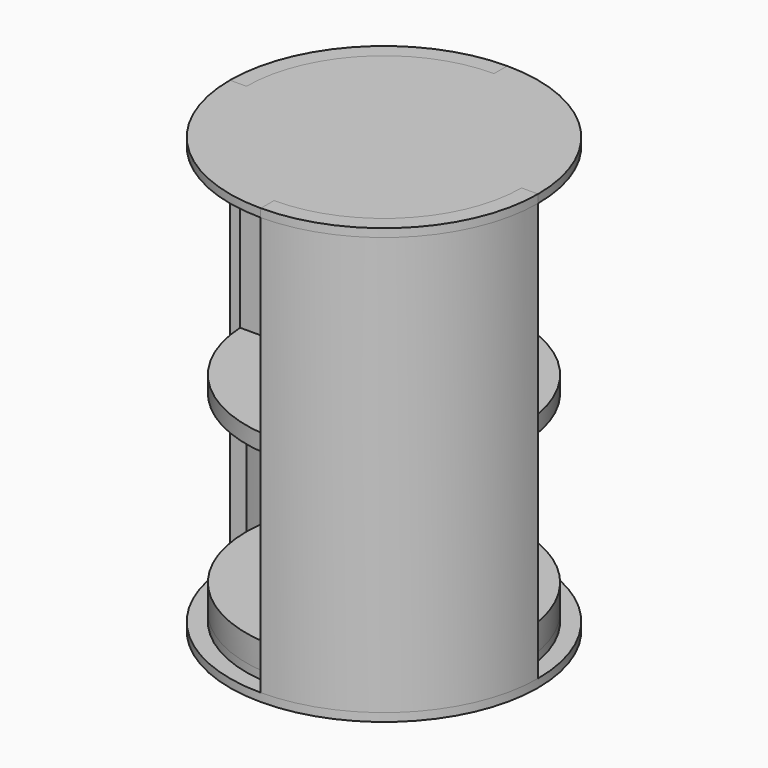
from build123d import *
from build123d import SkipClean  # not in build123d's __all__

# Parameters (mm, degrees)
F0_R      = 112
F1_DEPTH  = 6
F3_DEPTH  = 6
F5_DEPTH  = 140
F7_DEPTH  = 12
F9_DEPTH  = 140
F11_DEPTH = 6
F12_R     = 112
F12_R_2   = 100
F13_DEPTH = 6
F14_DEPTH = 25
F16_DEPTH = 310


with BuildPart() as f1:
    # F0 (on Top) → F1 (new body)
    with BuildSketch(Plane.XY):
        Circle(F0_R)
    extrude(amount=F1_DEPTH)

    # F2 (on face) → F3 (join)
    with BuildSketch(Plane.XY.offset(6)):
        with BuildLine():
            ThreePointArc((-100, 0), (0, -100), (100, 0))
            ThreePointArc((100, 0), (70.7106781187, 70.7106781187), (0, 100))
            ThreePointArc((0, 100), (-70.7106781187, 70.7106781187), (-100, 0))
        make_face()
    extrude(amount=F3_DEPTH)

    # F4 (on face) → F5 (join)
    with BuildSketch(Plane.XY.offset(12)):
        with BuildLine():
            ThreePointArc((6, 99.8198377077), (3.0013521308, 99.9549492791), (0, 100))
            ThreePointArc((0, 100), (-3.0013521308, 99.9549492791), (-6, 99.8198377077))
            Line((-6, 99.8198377077), (-6, -99.8198377077))
            ThreePointArc((-6, -99.8198377077), (-3.0013521308, -99.9549492791), (0, -100))
            ThreePointArc((0, -100), (3.0013521308, -99.9549492791), (6, -99.8198377077))
            Line((6, -99.8198377077), (6, 99.8198377077))
        make_face()
    extrude(amount=F5_DEPTH)

    # F6 (on face) → F7 (join)
    with BuildSketch(Plane.XY.offset(152)):
        with BuildLine():
            Line((-6, -99.8198377077), (-6, 99.8198377077))
            ThreePointArc((-6, 99.8198377077), (-100, 0), (-6, -99.8198377077))
        make_face()
        with BuildLine():
            Line((6, -99.8198377077), (6, 99.8198377077))
            ThreePointArc((6, 99.8198377077), (0, 100), (-6, 99.8198377077))
            Line((-6, 99.8198377077), (-6, -99.8198377077))
            ThreePointArc((-6, -99.8198377077), (0, -100), (6, -99.8198377077))
        make_face()
        with BuildLine():
            ThreePointArc((6, -99.8198377077), (72.8010988928, -68.556546004), (100, 0))
            ThreePointArc((100, 0), (72.8010988928, 68.556546004), (6, 99.8198377077))
            Line((6, 99.8198377077), (6, -99.8198377077))
        make_face()
    extrude(amount=F7_DEPTH)

    # F8 (on face) → F9 (join)
    with BuildSketch(Plane.XY.offset(164)):
        with BuildLine():
            Line((99.8198377077, 6), (-99.8198377077, 6))
            ThreePointArc((-99.8198377077, 6), (-99.9549492791, 3.0013521308), (-100, 0))
            ThreePointArc((-100, 0), (-99.9549492791, -3.0013521308), (-99.8198377077, -6))
            Line((-99.8198377077, -6), (99.8198377077, -6))
            ThreePointArc((99.8198377077, -6), (99.9549492791, -3.0013521308), (100, 0))
            ThreePointArc((100, 0), (99.9549492791, 3.0013521308), (99.8198377077, 6))
        make_face()
    extrude(amount=F9_DEPTH)

    # F10 (on face) → F11 (join)
    with BuildSketch(Plane.XY.offset(304)):
        with BuildLine():
            Line((-99.8198377077, 6), (99.8198377077, 6))
            ThreePointArc((99.8198377077, 6), (0, 100), (-99.8198377077, 6))
        make_face()
        with BuildLine():
            ThreePointArc((99.8198377077, -6), (99.9549492791, -3.0013521308), (100, 0))
            ThreePointArc((100, 0), (99.9549492791, 3.0013521308), (99.8198377077, 6))
            Line((99.8198377077, 6), (-99.8198377077, 6))
            ThreePointArc((-99.8198377077, 6), (-100, 0), (-99.8198377077, -6))
            Line((-99.8198377077, -6), (99.8198377077, -6))
        make_face()
        with BuildLine():
            ThreePointArc((-99.8198377077, -6), (0, -100), (99.8198377077, -6))
            Line((99.8198377077, -6), (-99.8198377077, -6))
        make_face()
    extrude(amount=F11_DEPTH)

    # F12 (on face) → F13 (join)
    with BuildSketch(Plane.XY.offset(310)):
        Circle(F12_R)
        Circle(F12_R_2, mode=Mode.SUBTRACT)
        Circle(F12_R_2)
    extrude(amount=F13_DEPTH)

    # F2 (on face) → F14 (join)
    with BuildSketch(Plane.XY.offset(6)):
        with BuildLine():
            ThreePointArc((-100, 0), (0, -100), (100, 0))
            ThreePointArc((100, 0), (70.7106781187, 70.7106781187), (0, 100))
            ThreePointArc((0, 100), (-70.7106781187, 70.7106781187), (-100, 0))
        make_face()
    with SkipClean():  # cleaning this boolean's faces spoils the solid; the shape is the same uncleaned
        extrude(amount=F14_DEPTH)

    # F15 (on face) → F16 (join)
    with BuildSketch(Plane.XY.offset(6)):
        with BuildLine():
            Line((0, 100), (0, 112))
            ThreePointArc((0, 112), (-79.1959594929, 79.1959594929), (-112, 0))
            Line((-112, 0), (-100, 0))
            ThreePointArc((-100, 0), (-70.7106781187, 70.7106781187), (0, 100))
        make_face()
        with BuildLine():
            ThreePointArc((0, -112), (79.1959594929, -79.1959594929), (112, 0))
            Line((112, 0), (100, 0))
            ThreePointArc((100, 0), (70.7106781187, -70.7106781187), (0, -100))
            Line((0, -100), (0, -112))
        make_face()
    extrude(amount=F16_DEPTH)


solid = f1.part
